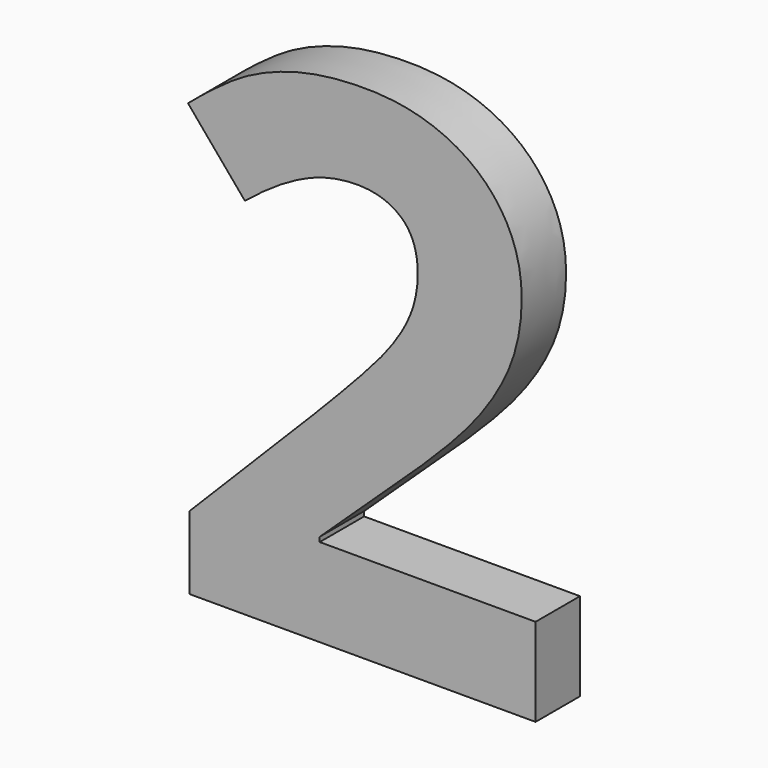
from build123d import *

# Parameters (mm, degrees)
F0_TEXT_SIZE = 62.5
F1_DEPTH     = 5


# Not quite as in the source:
# - Text() gives the source's letters only with a copy of the font that has no kerning and outlines rounded to 1/6400 em; it was checked with that copy


with BuildPart() as f1:
    # F0 (on Front) → F1 (new body)
    with BuildSketch(Plane.XZ):
        with Locations((-49.1015599385, 11.3671866462)):
            Text('2', F0_TEXT_SIZE, font='Open Sans', font_style=FontStyle.BOLD, text_align=(TextAlign.LEFT, TextAlign.BOTTOM))
    extrude(amount=F1_DEPTH)


solid = f1.part
